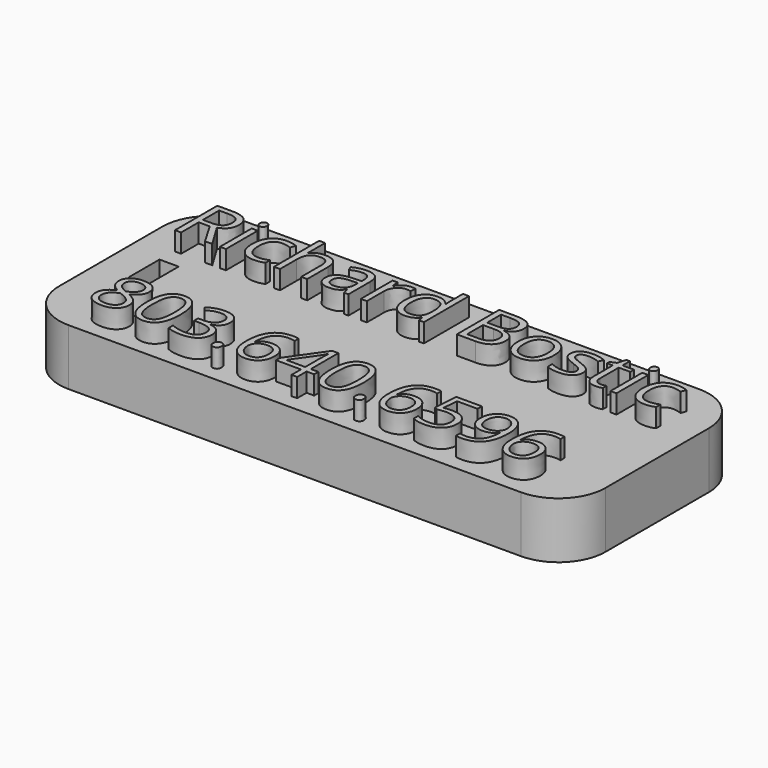
from build123d import *

# Parameters (mm, degrees)
F0_W         = 58.2218244672
F0_H         = 23.7748990767
F1_DEPTH     = 6
F2_R         = 5
F5_TEXT_SIZE = 7.6610389287
F4_TEXT_SIZE = 7.910581042
F6_DEPTH     = 2
F7_W         = 2.0408891141
F7_H         = 4.1555203497
F8_DEPTH     = 6


# Not quite as in the source:
# - Text() gives the source's letters only with a copy of the font that has no kerning and outlines rounded to 1/6400 em; it was checked with that copy


with BuildPart() as f1:
    # F0 (on Top) → F1 (new body)
    with BuildSketch(Plane.XY):
        Rectangle(F0_W, F0_H)
    extrude(amount=F1_DEPTH)

    # F2
    f2_edges = [f1.edges().sort_by_distance(p)[0] for p in [
        (-29.110912, 11.88745, 3),
        (29.110912, 11.88745, 3),
        (29.110912, -11.88745, 3),
        (-29.110912, -11.88745, 3),
    ]]
    fillet(f2_edges, radius=F2_R)

    # F5 (on face) + F4 (on face) → F6 (join)
    with BuildSketch(Plane.XY.offset(6)):
        with Locations((-24, -10.292549176)):
            Text('803.640.6596', F5_TEXT_SIZE, font='Open Sans', text_align=(TextAlign.LEFT, TextAlign.BOTTOM))
    with BuildSketch(Plane.XY.offset(6)):
        with Locations((-26.265601116, 4.0064482384)):
            Text('Richard Bostic', F4_TEXT_SIZE, font='Open Sans', text_align=(TextAlign.LEFT, TextAlign.BOTTOM))
    extrude(amount=F6_DEPTH)

    # F7 (on face) → F8 (cut, through all)
    with BuildSketch(Plane.XY.offset(6)):
        with Locations((-24.5690140873, 0)):
            Rectangle(F7_W, F7_H)
    extrude(amount=-F8_DEPTH, mode=Mode.SUBTRACT)


solid = f1.part
